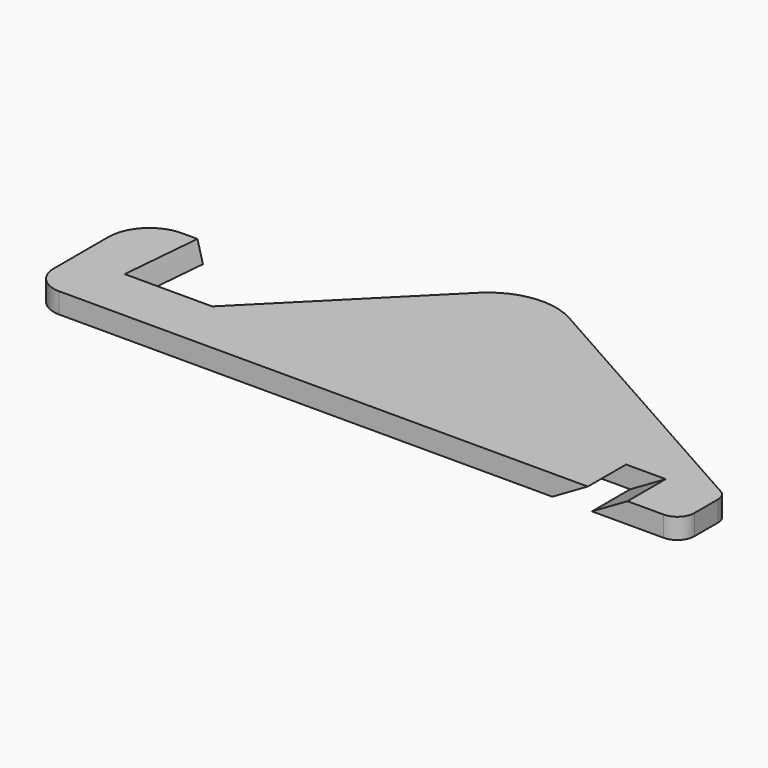
from build123d import *

# Parameters (mm, degrees)
F1_DEPTH = 3
F5_SIZE2 = 0.803838
F5_SIZE  = 2.99999
F4_W     = 7
F4_H     = 2.9
F6_DEPTH = 12.5


# Not quite as in the source:
# - a fillet or chamfer is up to 0.001 mm smaller than in the source, because OpenCascade refuses the exact size


with BuildPart() as f1:
    # F0 (on Top) → F1 (new body)
    with BuildSketch(Plane.XY):
        with BuildLine():
            Line((4, 0), (92.5, 0))
            ThreePointArc((92.5, 0), (94.267766953, 0.732233047), (95, 2.5))
            Line((95, 2.5), (95, 6.8303050312))
            ThreePointArc((95, 6.8303050312), (94.7264189756, 7.8399968261), (93.9805224793, 8.5734561054))
            Line((93.9805224793, 8.5734561054), (53.6105552952, 31.2815626464))
            ThreePointArc((53.6105552952, 31.2815626464), (47.3471346779, 32.4727846642), (41.636875087, 29.636875087))
            Line((41.636875087, 29.636875087), (20, 8))
            Line((20, 8), (8, 8))
            Line((8, 8), (9.0498639623, 20))
            Line((9.0498639623, 20), (6, 20))
            ThreePointArc((6, 20), (1.7573593129, 18.2426406871), (0, 14))
            Line((0, 14), (0, 4))
            ThreePointArc((0, 4), (1.1715728753, 1.1715728753), (4, 0))
        make_face()
    extrude(amount=F1_DEPTH)

    # F5 (size 3 and 0.8038475773 in the source; OpenCascade refuses exactly that, so slightly less here)
    f5_edges = [f1.edges().sort_by_distance(p)[0] for p in [
        (8.524932, 14, 3),
    ]]
    f5_side = f1.faces().sort_by_distance((8.524932, 14, 1.5))[0]
    chamfer(f5_edges, length=F5_SIZE, length2=F5_SIZE2, reference=f5_side)

    # F4 (on line) → F6 (cut, symmetric)
    with BuildSketch(Plane(origin=(61.5, 0, 35.5070415552), x_dir=(0, 1, 0), z_dir=(0.8660254038, 0, 0.5))):
        with Locations((3.5, -39.55)):
            Rectangle(F4_W, F4_H)
    extrude(amount=F6_DEPTH, both=True, mode=Mode.SUBTRACT)


solid = f1.part
